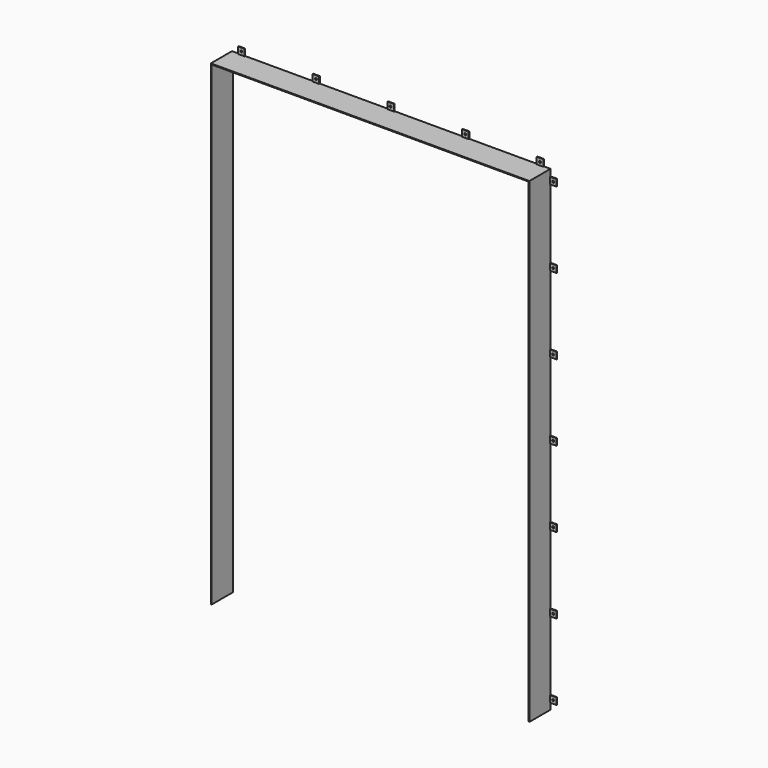
from build123d import *

# Parameters (mm, degrees)
F1_DEPTH = 101.6
F0_W     = 25.4
F0_H     = 25.4
F0_R     = 3.81
F2_DEPTH = 3.175


# Not quite as in the source:
# - a feature names something its author has since deleted; it is built from what else it names


with BuildPart() as f1:
    # F0 (on Front) → F1 (new body)
    with BuildSketch(Plane.XZ):
        Polygon((0, 25.4), (0, 0), (3.175, 0), (3.175, 1828.8), (1222.375, 1828.8), (1222.375, 0), (1225.55, 0), (1225.55, 25.4), (1225.55, 50.8), (1225.55, 318.0291666667), (1225.55, 343.4291666667), (1225.55, 610.6583333333), (1225.55, 636.0583333333), (1225.55, 903.2875), (1225.55, 928.6875), (1225.55, 1195.9166666667), (1225.55, 1221.3166666667), (1225.55, 1488.5458333333), (1225.55, 1513.9458333333), (1225.55, 1781.175), (1225.55, 1806.575), (1225.55, 1831.975), (1200.15, 1831.975), (1174.75, 1831.975), (912.8125, 1831.975), (887.4125, 1831.975), (625.475, 1831.975), (600.075, 1831.975), (338.1375, 1831.975), (312.7375, 1831.975), (50.8, 1831.975), (25.4, 1831.975), (0, 1831.975), (0, 1806.575), (0, 1781.175), (0, 1513.9458333333), (0, 1488.5458333333), (0, 1221.3166666667), (0, 1195.9166666667), (0, 928.6875), (0, 903.2875), (0, 636.0583333333), (0, 610.6583333333), (0, 343.4291666667), (0, 318.0291666667), (0, 50.8), align=None)
    extrude(amount=F1_DEPTH)

    # F0 (on Front) → F2 (join)
    with BuildSketch(Plane.XZ):
        with Locations((-12.7, 38.1)):
            Rectangle(F0_W, F0_H)
        with Locations((-12.7, 38.1)):
            Circle(F0_R, mode=Mode.SUBTRACT)
        with Locations((-12.7, 330.7291666667)):
            Rectangle(F0_W, F0_H)
        with Locations((-12.7, 330.7291666667)):
            Circle(F0_R, mode=Mode.SUBTRACT)
        with Locations((-12.7, 623.3583333333)):
            Rectangle(F0_W, F0_H)
        with Locations((-12.7, 623.3583333333)):
            Circle(F0_R, mode=Mode.SUBTRACT)
        with Locations((1238.25, 38.1)):
            Rectangle(F0_W, F0_H)
        with Locations((1238.25, 38.1)):
            Circle(F0_R, mode=Mode.SUBTRACT)
        with Locations((-12.7, 915.9875)):
            Rectangle(F0_W, F0_H)
        with Locations((-12.7, 915.9875)):
            Circle(F0_R, mode=Mode.SUBTRACT)
        with Locations((1238.25, 330.7291666667)):
            Rectangle(F0_W, F0_H)
        with Locations((1238.25, 330.7291666667)):
            Circle(F0_R, mode=Mode.SUBTRACT)
        with Locations((-12.7, 1208.6166666667)):
            Rectangle(F0_W, F0_H)
        with Locations((-12.7, 1208.6166666667)):
            Circle(F0_R, mode=Mode.SUBTRACT)
        with Locations((1238.25, 623.3583333333)):
            Rectangle(F0_W, F0_H)
        with Locations((1238.25, 623.3583333333)):
            Circle(F0_R, mode=Mode.SUBTRACT)
        with Locations((-12.7, 1501.2458333333)):
            Rectangle(F0_W, F0_H)
        with Locations((-12.7, 1501.2458333333)):
            Circle(F0_R, mode=Mode.SUBTRACT)
        with Locations((1238.25, 915.9875)):
            Rectangle(F0_W, F0_H)
        with Locations((1238.25, 915.9875)):
            Circle(F0_R, mode=Mode.SUBTRACT)
        with Locations((-12.7, 1793.875)):
            Rectangle(F0_W, F0_H)
        with Locations((-12.7, 1793.875)):
            Circle(F0_R, mode=Mode.SUBTRACT)
        with Locations((1238.25, 1208.6166666667)):
            Rectangle(F0_W, F0_H)
        with Locations((1238.25, 1208.6166666667)):
            Circle(F0_R, mode=Mode.SUBTRACT)
        with Locations((38.1, 1844.675)):
            Rectangle(F0_W, F0_H)
        with Locations((38.1, 1844.675)):
            Circle(F0_R, mode=Mode.SUBTRACT)
        with Locations((1238.25, 1501.2458333333)):
            Rectangle(F0_W, F0_H)
        with Locations((1238.25, 1501.2458333333)):
            Circle(F0_R, mode=Mode.SUBTRACT)
        with Locations((325.4375, 1844.675)):
            Rectangle(F0_W, F0_H)
        with Locations((325.4375, 1844.675)):
            Circle(F0_R, mode=Mode.SUBTRACT)
        with Locations((1238.25, 1793.875)):
            Rectangle(F0_W, F0_H)
        with Locations((1238.25, 1793.875)):
            Circle(F0_R, mode=Mode.SUBTRACT)
        with Locations((612.775, 1844.675)):
            Rectangle(F0_W, F0_H)
        with Locations((612.775, 1844.675)):
            Circle(F0_R, mode=Mode.SUBTRACT)
        with Locations((1187.45, 1844.675)):
            Rectangle(F0_W, F0_H)
        with Locations((1187.45, 1844.675)):
            Circle(F0_R, mode=Mode.SUBTRACT)
        with Locations((900.1125, 1844.675)):
            Rectangle(F0_W, F0_H)
        with Locations((900.1125, 1844.675)):
            Circle(F0_R, mode=Mode.SUBTRACT)
    extrude(amount=F2_DEPTH)


solid = f1.part
